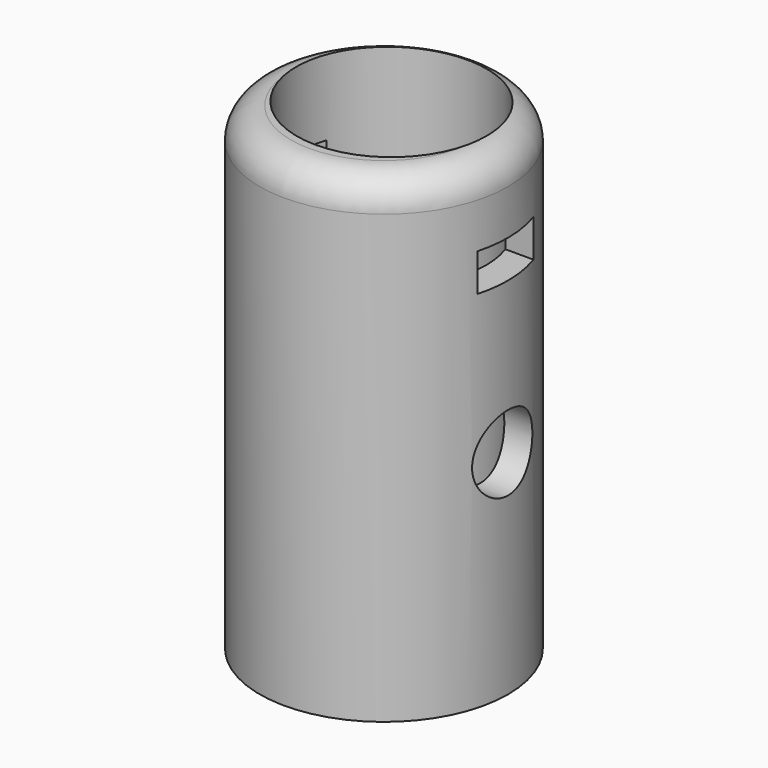
from build123d import *

# Parameters (mm, degrees)
F0_R          = 20
F0_R_2        = 15.237
F1_DEPTH      = 77
F3_R          = 6.065714741
F4_DEPTH      = 25
F4_DEPTH_BACK = 25
F3_W          = 11.689950712
F3_H          = 6.0669332743
F5_DEPTH      = 25
F5_DEPTH_BACK = 25


# Not quite as in the source:
# - a fillet or chamfer that OpenCascade refuses, or shapes differently, is made with other operations: its cross-section is extruded or revolved along the edge and cut away or added


with BuildPart() as f1:
    # F0 (on Top) → F1 (new body)
    with BuildSketch(Plane.XY):
        Circle(F0_R)
        with Locations((0, 1.5118854353)):
            Circle(F0_R_2, mode=Mode.SUBTRACT)
    extrude(amount=F1_DEPTH)

    # F2: fillet of radius 5 on 1 edges, made by hand

    # F2_s1 → F2_t2 (revolve, cut)
    with BuildSketch(Plane.XZ):
        with BuildLine():
            ThreePointArc((20, 72), (18.5355339059, 75.5355339059), (15, 77))
            Line((15, 77), (20, 77))
            Line((20, 77), (20, 72))
        make_face()
    revolve(axis=Axis((0, 0, 77), (0, 0, 1)), mode=Mode.SUBTRACT)

    # F3 (on Right) → F4 (join, two sides)
    with BuildSketch(Plane.YZ) as f4_sk:
        with Locations((0, 34.2814810574)):
            Circle(F3_R)
    extrude(amount=F4_DEPTH)
    extrude(f4_sk.sketch, amount=-F4_DEPTH_BACK)

    # F3 (on Right) → F5 (cut, two sides)
    with BuildSketch(Plane.YZ) as f5_sk:
        with Locations((0, 34.2814810574)):
            Circle(F3_R)
        with Locations((0.5918950774, 61.7306679487)):
            Rectangle(F3_W, F3_H)
    extrude(amount=-F5_DEPTH, mode=Mode.SUBTRACT)
    extrude(f5_sk.sketch, amount=F5_DEPTH_BACK, mode=Mode.SUBTRACT)


solid = f1.part
